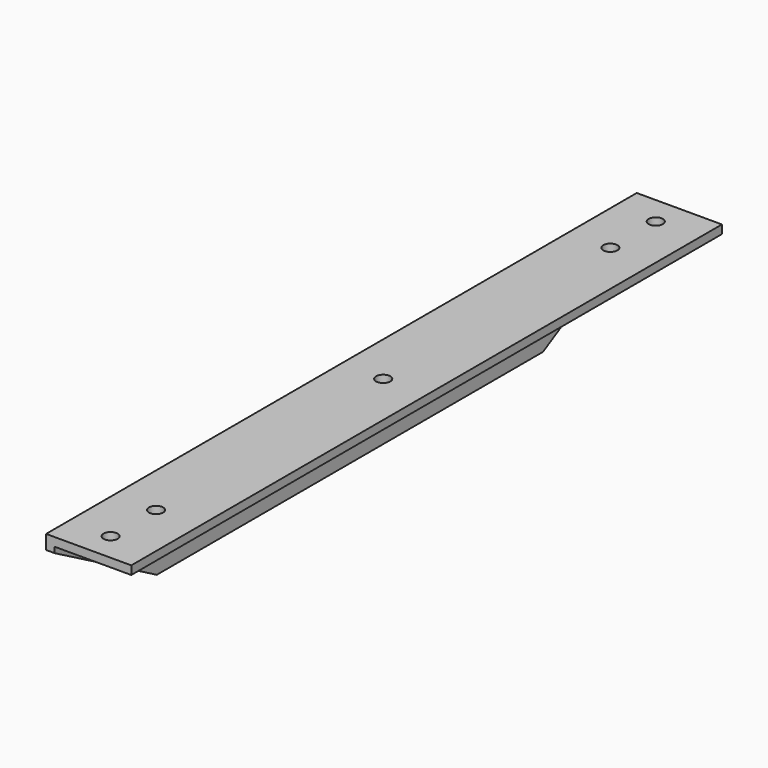
from build123d import *

# Parameters (mm, degrees)
F1_DEPTH = 130
F3_D     = 7
F5_D     = 5
F7_DEPTH = 25


# Not quite as in the source:
# - a feature names something its author has since deleted; it is built from what else it names


with BuildPart() as f1:
    # F0 (on Front) → F1 (new body, symmetric)
    with BuildSketch(Plane.XZ):
        Polygon((0, 30), (0, 0), (3, 0), (3, 27), (30, 27), (30, 30), align=None)
    extrude(amount=F1_DEPTH, both=True)

    # F3 (through all)
    with Locations(Plane(origin=(0, 0, 0), x_dir=(0, -1, 0), z_dir=(-1, 0, 0))):
        with Locations((-31.5, 10), (31.5, 10)):
            Hole(F3_D / 2)

    # F5 (through all)
    with Locations(Plane.XY.offset(30)):
        with Locations((14.7187495604, 0), (14.7187495604, -100), (14.7187495604, 100), (14.7187495604, -120), (14.7187495604, 120)):
            Hole(F5_D / 2)

    # F6 (on face) → F7 (cut)
    with BuildSketch(Plane(origin=(0, 0, 0), x_dir=(0, -1, 0), z_dir=(-1, 0, 0))):
        Polygon((-85, 0), (-130, 25), (-130, 0), align=None)
        Polygon((130, 0), (130, 25), (85, 0), align=None)
    extrude(amount=-F7_DEPTH, mode=Mode.SUBTRACT)


solid = f1.part
